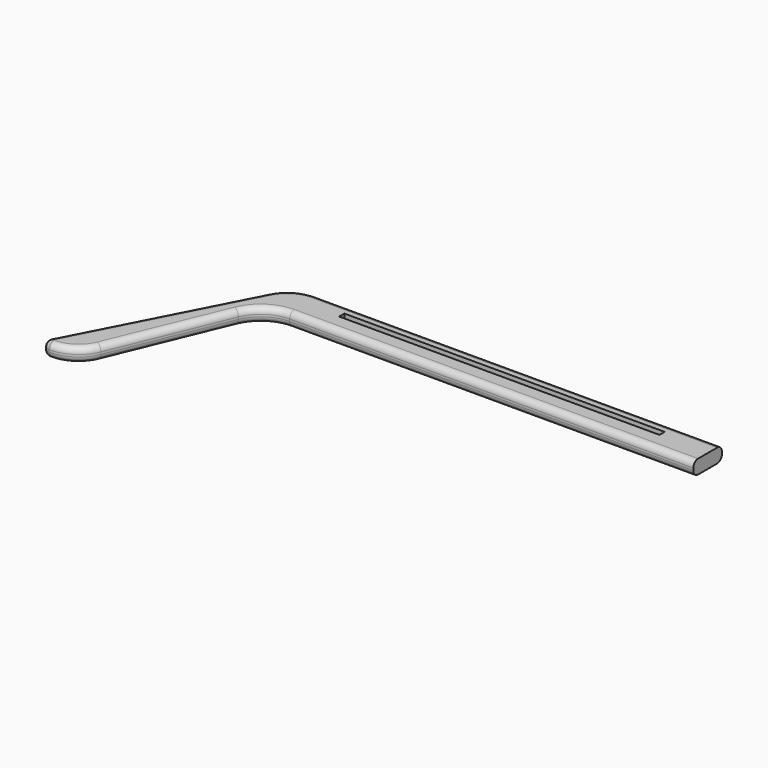
from build123d import *

# Parameters (mm, degrees)
F0_W         = 73.972383514
F0_H         = 1.5005278401
F1_DEPTH     = 3.25
F2_R         = 1.375
F3_R         = 1.375
F4_T1_DEPTH  = 42.9737045288
F4_T3_DEPTH  = 0.5
F4_T5_DEPTH  = 97.1535263256
F4_T10_DEPTH = 1.375
F4_T16_DEPTH = 1.375
F4_T20_ANGLE = 62.6710528925
F4_T22_ANGLE = 62.6710528925


# Not quite as in the source:
# - a fillet or chamfer that OpenCascade refuses, or shapes differently, is made with other operations: its cross-section is extruded or revolved along the edge and cut away or added


with BuildPart() as f1:
    # F0 (on Top) → F1 (new body)
    with BuildSketch(Plane.XY):
        with BuildLine():
            Line((62.3850544982, 0), (62.3850544982, 8.25))
            Line((62.3850544982, 8.25), (-31.3309718274, 8.25))
            ThreePointArc((-31.3309718274, 8.25), (-35.6733794922, 7.0320400779), (-38.7489899112, 3.7334720175))
            Line((-38.7489899112, 3.7334720175), (-59.5149430004, -36.45))
            Line((-59.5149430004, -36.45), (-57.0939640871, -36.45))
            ThreePointArc((-57.0939640871, -36.45), (-52.4551081593, -35.0428751739), (-49.3797131513, -31.2957522588))
            Line((-49.3797131513, -31.2957522588), (-38.5501753509, -5.1542477412))
            ThreePointArc((-38.5501753509, -5.1542477412), (-35.474780343, -1.4071248261), (-30.8359244151, 0))
            Line((-30.8359244151, 0), (62.3850544982, 0))
        make_face()
        with Locations((14.1874579713, 4.9997360799)):
            Rectangle(F0_W, F0_H, mode=Mode.SUBTRACT)
    extrude(amount=F1_DEPTH)

    # F2
    f2_edges = [f1.edges().sort_by_distance(p)[0] for p in [
        (15.774565, 0, 3.25),
    ]]
    fillet(f2_edges, radius=F2_R)

    # F3
    f3_edges = [f1.edges().sort_by_distance(p)[0] for p in [
        (15.774565, 0, 0),
    ]]
    fillet(f3_edges, radius=F3_R)

    # F4: fillet of radius 1.375 on 2 edges, made by hand

    # F4_s2 → F4_t1 (cut)
    with BuildSketch(Plane(origin=(-6.6444578792, -12.8574588468, 0), x_dir=(0, 0, 1), z_dir=(-0.4590984452, -0.8883853993, 0))):
        with BuildLine():
            ThreePointArc((1.375, 36.1380680715), (0.4027281759, 35.7353398956), (0, 34.7630680715))
            Line((0, 34.7630680715), (0, 36.1380680715))
            Line((0, 36.1380680715), (1.375, 36.1380680715))
        make_face()
        with BuildLine():
            ThreePointArc((1.875, 36.1380680715), (2.8472718241, 35.7353398956), (3.25, 34.7630680715))
            Line((3.25, 34.7630680715), (3.25, 36.1380680715))
            Line((3.25, 36.1380680715), (1.875, 36.1380680715))
        make_face()
    extrude(amount=F4_T1_DEPTH, mode=Mode.SUBTRACT)

    # F4_s4 → F4_t3 (cut)
    with BuildSketch(Plane.XY.offset(1.375)):
        with BuildLine():
            ThreePointArc((-58.478150845, -34.4437396378), (-58.4310586584, -35.7900671304), (-57.256620921, -36.45))
            Line((-57.256620921, -36.45), (-59.5149430004, -36.45))
            Line((-59.5149430004, -36.45), (-58.478150845, -34.4437396378))
        make_face()
    extrude(amount=F4_T3_DEPTH, mode=Mode.SUBTRACT)

    # F4_s6 → F4_t5 (cut)
    with BuildSketch(Plane.YZ.offset(-31.3309718274)):
        with BuildLine():
            ThreePointArc((6.875, 3.25), (7.8472718241, 2.8472718241), (8.25, 1.875))
            Line((8.25, 1.875), (8.25, 3.25))
            Line((8.25, 3.25), (6.875, 3.25))
        make_face()
        with BuildLine():
            ThreePointArc((6.875, 0), (7.8472718241, 0.4027281759), (8.25, 1.375))
            Line((8.25, 1.375), (8.25, 0))
            Line((8.25, 0), (6.875, 0))
        make_face()
    extrude(amount=F4_T5_DEPTH, mode=Mode.SUBTRACT)


with BuildPart() as f4_tool8:
    # F4_s9 → F4_t10 (new body)
    with BuildSketch(Plane.XY.offset(1.875)):
        Polygon((-57.256620921, -35.075), (-58.478150845, -34.4437396378), (-59.5149430004, -36.45), (-57.256620921, -36.45), align=None)
    extrude(amount=F4_T10_DEPTH)

    # F4_s11 → F4_t12 (revolve, cut)
    with BuildSketch(Plane(origin=(-57.256620921, -35.075, 1.875), x_dir=(0.8541365363, 0.5200488221, 0), z_dir=(0.5200488221, -0.8541365363, 0))):
        with BuildLine():
            ThreePointArc((0, -1.375), (1.375, 0), (0, 1.375))
            Line((0, 1.375), (0, -1.375))
        make_face()
    revolve(axis=Axis((-57.256620921, -35.075, 1.875), (0, 0, 1)), mode=Mode.SUBTRACT)


with BuildPart() as f1_1:
    add(f1.part)

    # F4_t7: cut F4_tool8
    add(f4_tool8.part, mode=Mode.SUBTRACT)


with BuildPart() as f4_tool14:
    # F4_s15 → F4_t16 (new body)
    with BuildSketch(Plane.XY.offset(1.375)):
        Polygon((-57.256620921, -35.075), (-58.478150845, -34.4437396378), (-59.5149430004, -36.45), (-57.256620921, -36.45), align=None)
    extrude(amount=-F4_T16_DEPTH)

    # F4_s17 → F4_t18 (revolve, cut)
    with BuildSketch(Plane(origin=(-57.256620921, -35.075, 1.375), x_dir=(0.8541365363, 0.5200488221, 0), z_dir=(-0.5200488221, 0.8541365363, 0))):
        with BuildLine():
            ThreePointArc((0, -1.375), (1.375, 0), (0, 1.375))
            Line((0, 1.375), (0, -1.375))
        make_face()
    revolve(axis=Axis((-57.256620921, -35.075, 1.375), (0, 0, -1)), mode=Mode.SUBTRACT)


with BuildPart() as f1_2:
    add(f1_1.part)

    # F4_t13: cut F4_tool14
    add(f4_tool14.part, mode=Mode.SUBTRACT)

    # F4_s19 → F4_t20 (revolve, cut)
    with BuildSketch(Plane.YZ.offset(-31.3309718274)):
        with BuildLine():
            ThreePointArc((6.875, 3.25), (7.8472718241, 2.8472718241), (8.25, 1.875))
            Line((8.25, 1.875), (8.25, 3.25))
            Line((8.25, 3.25), (6.875, 3.25))
        make_face()
    revolve(axis=Axis((-31.3309718274, -0.1, 3.25), (0, 0, 1)), revolution_arc=F4_T20_ANGLE, mode=Mode.SUBTRACT)

    # F4_s21 → F4_t22 (revolve, cut)
    with BuildSketch(Plane.YZ.offset(-31.3309718274)):
        with BuildLine():
            ThreePointArc((6.875, 0), (7.8472718241, 0.4027281759), (8.25, 1.375))
            Line((8.25, 1.375), (8.25, 0))
            Line((8.25, 0), (6.875, 0))
        make_face()
    revolve(axis=Axis((-31.3309718274, -0.1, 0), (0, 0, 1)), revolution_arc=F4_T22_ANGLE, mode=Mode.SUBTRACT)


solid = f1_2.part
